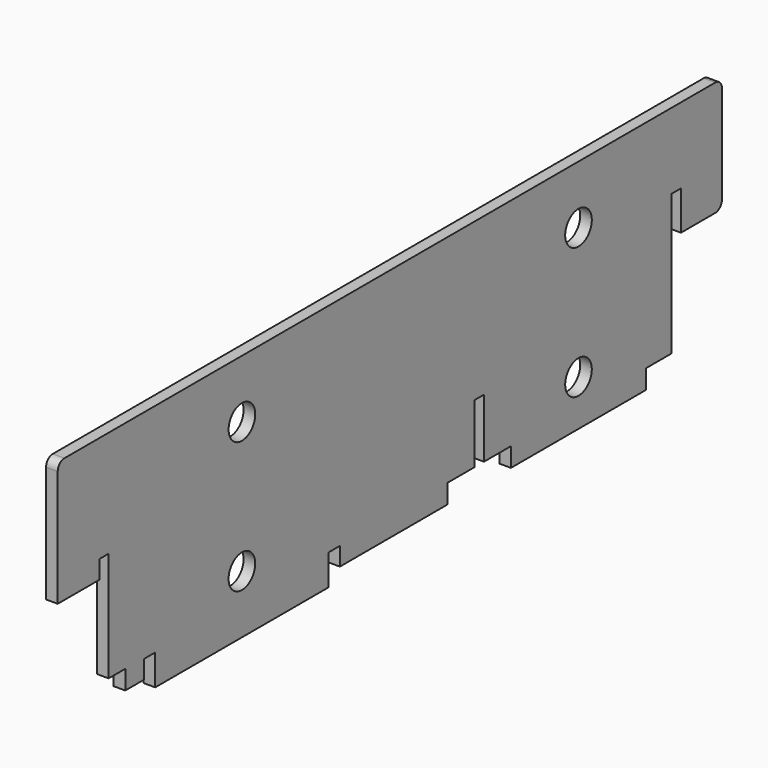
from build123d import *

# Parameters (mm, degrees)
F0_R     = 2
F1_DEPTH = 1.4
F2_R     = 1


with BuildPart() as f1:
    # F0 (on Right) → F1 (new body)
    with BuildSketch(Plane.YZ):
        Polygon((-35.25, -14.9), (-9.2, -14.9), (-9.2, -13.4), (-9.2, -11.2), (-7.5, -11.2), (-7.5, -13.4), (8.7, -13.4), (8.7, -11.1), (12.75, -11.1), (12.75, -4), (14.15, -4), (14.15, -11.1), (18.2, -11.1), (18.2, -13.4), (38.5, -13.4), (38.5, -11.1), (42.35, -11.1), (42.35, 5.8), (43.75, 5.8), (43.75, 1.1), (49.9, 1.1), (49.9, 14.9), (-49.9, 14.9), (-49.9, 6.4402827993), (-49.9, 2.1), (-49.9, -0.1), (-43.65, -0.1), (-43.65, 2.1), (-42.25, 2.1), (-42.25, -11.1), (-39.75, -11.1), (-39.75, -13.4), (-36.95, -13.4), (-36.95, -11.2), (-35.25, -11.2), (-35.25, -13.4), align=None)
        with Locations((-22.225, -7.9)):
            Circle(F0_R, mode=Mode.SUBTRACT)
        with Locations((28.35, -7.9)):
            Circle(F0_R, mode=Mode.SUBTRACT)
        with Locations((-22.225, 7.9)):
            Circle(F0_R, mode=Mode.SUBTRACT)
        with Locations((28.35, 7.9)):
            Circle(F0_R, mode=Mode.SUBTRACT)
    extrude(amount=F1_DEPTH)

    # F2
    f2_edges = [f1.edges().sort_by_distance(p)[0] for p in [
        (0.7, -49.9, 14.9),
        (0.7, 49.9, 14.9),
        (0.7, 49.9, 1.1),
    ]]
    fillet(f2_edges, radius=F2_R)


solid = f1.part
